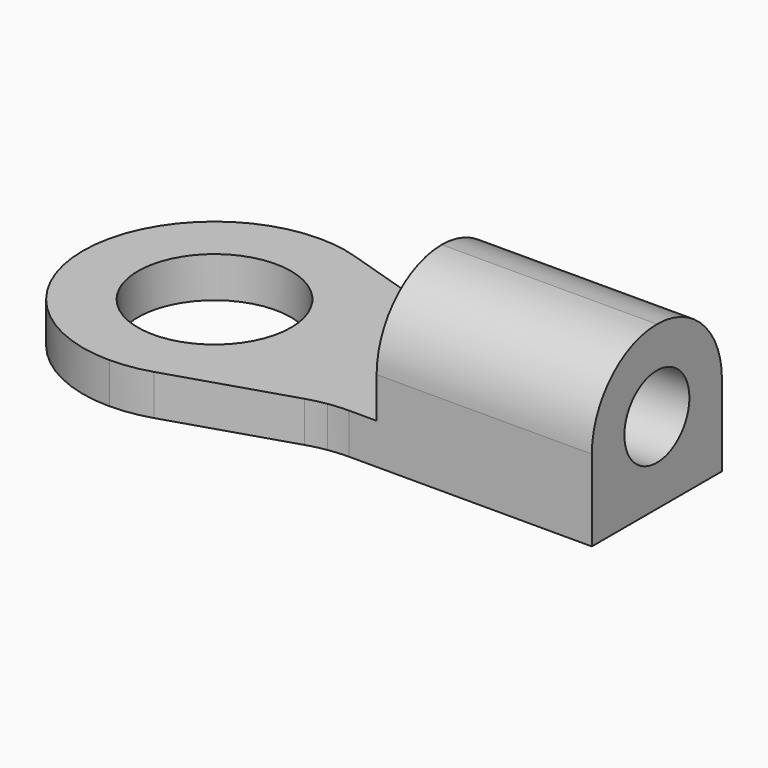
from build123d import *

# Parameters (mm, degrees)
F0_R     = 1.6
F1_DEPTH = 0.85
F2_W     = 4.5
F2_H     = 3.4
F3_DEPTH = 2.55
F4_R     = 1.69999
F5_R     = 0.85
F6_DEPTH = 25


# Not quite as in the source:
# - a fillet or chamfer is up to 0.001 mm smaller than in the source, because OpenCascade refuses the exact size


with BuildPart() as f1:
    # F0 (on Top) → F1 (new body)
    with BuildSketch(Plane.XY):
        with BuildLine():
            Line((6.9237405853, 1.05), (12, 1.05))
            Line((12, 1.05), (12, 4.45))
            Line((12, 4.45), (6.9237405853, 4.45))
            ThreePointArc((6.9237405853, 4.45), (6.7112348648, 4.4582229633), (6.5, 4.4828426773))
            ThreePointArc((6.5, 4.4828426773), (6.2961678451, 4.5225660688), (6.0959144518, 4.5775576474))
            Line((6.0959144518, 4.5775576474), (3.5778261335, 5.3724423526))
            ThreePointArc((3.5778261335, 5.3724423526), (3.1687980004, 5.4679235153), (2.75, 5.5))
            ThreePointArc((2.75, 5.5), (0.8054563517, 4.6945436483), (0, 2.75))
            ThreePointArc((0, 2.75), (0.8054563517, 0.8054563517), (2.75, 0))
            ThreePointArc((2.75, 0), (3.1687980004, 0.0320764847), (3.5778261335, 0.1275576474))
            Line((3.5778261335, 0.1275576474), (6.0959144518, 0.9224423526))
            ThreePointArc((6.0959144518, 0.9224423526), (6.2961678451, 0.9774339312), (6.5, 1.0171573227))
            ThreePointArc((6.5, 1.0171573227), (6.7112348648, 1.0417770367), (6.9237405853, 1.05))
        make_face()
        with Locations((2.75, 2.75)):
            Circle(F0_R, mode=Mode.SUBTRACT)
    extrude(amount=F1_DEPTH)

    # F2 (on face) → F3 (join)
    with BuildSketch(Plane.XY.offset(0.85)):
        with Locations((9.75, 2.75)):
            Rectangle(F2_W, F2_H)
    extrude(amount=F3_DEPTH)

    # F4 (radius 1.7 in the source; OpenCascade refuses exactly that, so slightly less here)
    f4_edges = [f1.edges().sort_by_distance(p)[0] for p in [
        (9.75, 4.45, 3.4),
        (9.75, 1.05, 3.4),
    ]]
    fillet(f4_edges, radius=F4_R)

    # F5 (on face) → F6 (cut)
    with BuildSketch(Plane.YZ.offset(12)):
        with Locations((2.75, 1.7)):
            Circle(F5_R)
    extrude(amount=-F6_DEPTH, mode=Mode.SUBTRACT)


solid = f1.part
